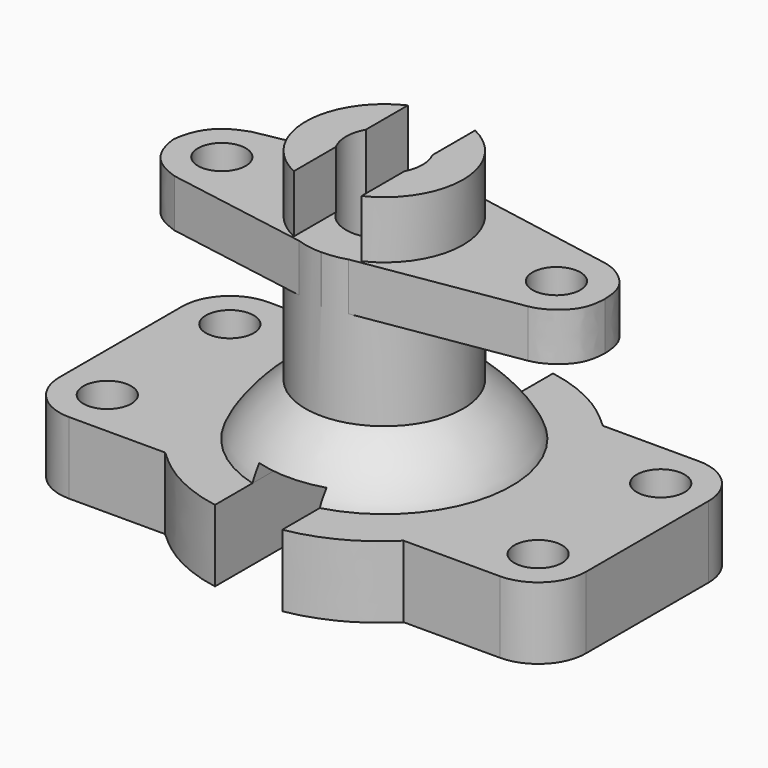
from build123d import *

# Parameters (mm, degrees)
F1_DEPTH  = 150
F2_R      = 100
F3_R      = 100
F4_R      = 100
F5_R      = 100
F6_R      = 50
F6_W      = 140.4859647155
F6_H      = 520
F6_H_2    = 39.2821230811
F6_H_3    = 46.7312682828
F7_DEPTH  = 150
F11_DEPTH = 30
F12_W     = 140.4859647155
F12_H     = 552.6287908551
F12_H_2   = 21.1866145137
F13_DEPTH = 25
F14_R     = 164.5018596362
F15_DEPTH = 500
F16_W     = 140.9460157156
F16_H     = 576.6842067242
F17_DEPTH = 120
F19_DEPTH = 100
F20_R     = 50
F21_DEPTH = 100
F22_R     = 80
F23_DEPTH = 600


with BuildPart() as f1:
    # F0 (on Top) → F1 (new body)
    with BuildSketch(Plane.XY):
        Polygon((-255.04347682, 304.850508936), (-555.8274231851, 304.850508936), (-555.8274231851, -215.149491064), (-255.04347682, -215.149491064), (-76.0704055429, -215.149491064), (64.4155591726, -215.149491064), (243.3886304498, -215.149491064), (544.1725768149, -215.149491064), (544.1725768149, 304.850508936), (243.3886304498, 304.850508936), (64.4155591726, 304.850508936), (-76.0704055429, 304.850508936), align=None)
        with BuildLine():
            add(Edge.make_bspline(
                [(-76.0704055429, 398.3130455017), (-111.1650615931, 392.6026821136), (-174.2262606106, 368.6970989499), (-217.5068408251, 339.1989171505), (-255.04347682, 304.850508936)],
                knots=[0, 0, 0, 0, 0.4864834978, 1, 1, 1, 1], degree=3))
            Line((-255.04347682, 304.850508936), (-76.0704055429, 304.850508936))
            Line((-76.0704055429, 304.850508936), (-76.0704055429, 398.3130455017))
        make_face()
        with BuildLine():
            Line((-76.0704055429, -215.149491064), (-255.04347682, -215.149491064))
            add(Edge.make_bspline(
                [(-76.0704055429, -308.6120276296), (-111.1650615931, -302.9016642416), (-174.2262606106, -278.9960810778), (-217.5068408251, -249.4978992784), (-255.04347682, -215.149491064)],
                knots=[0, 0, 0, 0, 0.4864834978, 1, 1, 1, 1], degree=3))
            Line((-76.0704055429, -308.6120276296), (-76.0704055429, -215.149491064))
        make_face()
        with BuildLine():
            Line((64.4155591726, 398.3130455017), (64.4155591726, 304.850508936))
            Line((64.4155591726, 304.850508936), (243.3886304498, 304.850508936))
            add(Edge.make_bspline(
                [(64.4155591726, 398.3130455017), (99.5102152228, 392.6026821136), (162.5714142404, 368.6970989499), (205.8519944549, 339.1989171505), (243.3886304498, 304.850508936)],
                knots=[0, 0, 0, 0, 0.4864834978, 1, 1, 1, 1], degree=3))
        make_face()
        with BuildLine():
            Line((243.3886304498, -215.149491064), (64.4155591726, -215.149491064))
            Line((64.4155591726, -215.149491064), (64.4155591726, -308.6120276296))
            add(Edge.make_bspline(
                [(64.4155591726, -308.6120276296), (99.5102152228, -302.9016642416), (162.5714142404, -278.9960810778), (205.8519944549, -249.4978992784), (243.3886304498, -215.149491064)],
                knots=[0, 0, 0, 0, 0.4864834978, 1, 1, 1, 1], degree=3))
        make_face()
    extrude(amount=F1_DEPTH)

    # F2
    f2_edges = [f1.edges().sort_by_distance(p)[0] for p in [
        (-555.827423, -215.149491, 75),
    ]]
    fillet(f2_edges, radius=F2_R)

    # F3
    f3_edges = [f1.edges().sort_by_distance(p)[0] for p in [
        (-555.827423, 304.850509, 75),
    ]]
    fillet(f3_edges, radius=F3_R)

    # F4
    f4_edges = [f1.edges().sort_by_distance(p)[0] for p in [
        (544.172577, 304.850509, 75),
    ]]
    fillet(f4_edges, radius=F4_R)

    # F5
    f5_edges = [f1.edges().sort_by_distance(p)[0] for p in [
        (544.172577, -215.149491, 75),
    ]]
    fillet(f5_edges, radius=F5_R)

    # F6 (on face) → F7 (cut)
    with BuildSketch(Plane.XY.offset(150)):
        with Locations((-455.8274231851, -115.149491064)):
            Circle(F6_R)
        with Locations((-455.8274231851, 204.850508936)):
            Circle(F6_R)
        with Locations((444.1725768149, 204.850508936)):
            Circle(F6_R)
        with Locations((444.1725768149, -115.149491064)):
            Circle(F6_R)
        with Locations((-5.8274231851, 44.850508936)):
            Rectangle(F6_W, F6_H)
        with Locations((-5.8274231851, 324.4915704766)):
            Rectangle(F6_W, F6_H_2)
        with Locations((-5.8274231851, -238.5151252054)):
            Rectangle(F6_W, F6_H_3)
    extrude(amount=-F7_DEPTH, mode=Mode.SUBTRACT)


with BuildPart() as f10:
    # F9 (on offset) → F10 (revolve)
    with BuildSketch(Plane.XZ.offset(-46)):
        with BuildLine():
            add(Edge.make_bspline(
                [(-170.576184988, 258.8557302952), (-198.9692002535, 247.1876442432), (-258.6858570576, 186.6178661585), (-272.3354101181, 149.9347686768)],
                knots=[0, 0, 0, 0, 149.0594370678, 149.0594370678, 149.0594370678, 149.0594370678], degree=3))
            Line((-272.3354101181, 149.9347686768), (-6.1521544121, 149.9347686768))
            Line((-6.1521544121, 149.9347686768), (-6.1521544121, 258.8557302952))
            Line((-6.1521544121, 258.8557302952), (-170.576184988, 258.8557302952))
        make_face()
    revolve(axis=Axis((-6.1521544121, 46, 204.395249486), (0, 0, 1)))

    # F6 (on face) → F11 (cut)
    with BuildSketch(Plane.XY.offset(150)):
        with Locations((-455.8274231851, -115.149491064)):
            Circle(F6_R)
        with Locations((-455.8274231851, 204.850508936)):
            Circle(F6_R)
        with Locations((444.1725768149, 204.850508936)):
            Circle(F6_R)
        with Locations((444.1725768149, -115.149491064)):
            Circle(F6_R)
        with Locations((-5.8274231851, 44.850508936)):
            Rectangle(F6_W, F6_H)
        with Locations((-5.8274231851, 324.4915704766)):
            Rectangle(F6_W, F6_H_2)
        with Locations((-5.8274231851, -238.5151252054)):
            Rectangle(F6_W, F6_H_3)
    extrude(amount=F11_DEPTH, mode=Mode.SUBTRACT)

    # F12 (on face) → F13 (cut)
    with BuildSketch(Plane.XY.offset(150)):
        with Locations((-5.8274231851, 56.1556639673)):
            Rectangle(F12_W, F12_H)
        with Locations((-5.8274231851, -230.7520387171)):
            Rectangle(F12_W, F12_H_2)
    extrude(amount=-F13_DEPTH, mode=Mode.SUBTRACT)

    # F14 (on face) → F15 (join)
    with BuildSketch(Plane(origin=(0, 0, 180), x_dir=(1, 0, 0), z_dir=(0, 0, -1))):
        with Locations((-6.1521544121, -46)):
            Circle(F14_R)
    extrude(amount=-F15_DEPTH)

    # F16 (on face) → F17 (cut)
    with BuildSketch(Plane.XY.offset(680)):
        with Locations((-5.5357143283, 38.3945852518)):
            Rectangle(F16_W, F16_H)
    extrude(amount=-F17_DEPTH, mode=Mode.SUBTRACT)

    # F18 (on face) → F19 (join)
    with BuildSketch(Plane.XY.offset(560)):
        with BuildLine():
            ThreePointArc((-76.0087221861, 194.932608124), (-71.1586390109, 197.1126029949), (-66.2406310646, 199.13470148))
            Line((-66.2406310646, 199.13470148), (-361.811041832, 142.5854861736))
            add(Edge.make_bspline(
                [(-361.811041832, 142.5854861736), (-379.9521342538, 136.153064008), (-417.6021453447, 119.6618540034), (-440.2464032173, 76.1652365327), (-443.6650574207, 42.4059182405)],
                knots=[0, 0, 0, 0, 0.4563088796, 1, 1, 1, 1], degree=3))
            add(Edge.make_bspline(
                [(-361.811041832, -57.7736496925), (-379.9521342538, -51.3412275269), (-417.6021453447, -34.8500175223), (-440.2464032173, 8.6465999484), (-443.6650574207, 42.4059182405)],
                knots=[0, 0, 0, 0, 0.4563088796, 1, 1, 1, 1], degree=3))
            Line((-361.811041832, -57.7736496925), (-60.1914490263, -109.3725087053))
            ThreePointArc((-60.1914490263, -109.3725087053), (-68.183712986, -106.3579586523), (-76.0087221861, -102.932608124))
            Line((-76.0087221861, -102.932608124), (-76.0087221861, 194.932608124))
        make_face()
        with BuildLine():
            Line((376.153409481, 141.4481401443), (50.8522174401, 200.3093108452))
            ThreePointArc((50.8522174401, 200.3093108452), (57.9640739697, 197.4924786313), (64.9372935295, 194.348077895))
            Line((64.9372935295, 194.348077895), (64.9372935295, -102.348077895))
            ThreePointArc((64.9372935295, -102.348077895), (54.9647832463, -106.7271480616), (44.724353476, -110.4367053121))
            Line((44.724353476, -110.4367053121), (376.153409481, -57.1924522519))
            add(Edge.make_bspline(
                [(376.153409481, -57.1924522519), (401.8360972404, -52.8410449624), (444.3782155693, -22.4764027045), (456.7823708057, 10.2454349399), (458.1390619278, 42.1278439462)],
                knots=[0, 0, 0, 0, 0.5069670176, 1, 1, 1, 1], degree=3))
            add(Edge.make_bspline(
                [(376.153409481, 141.4481401443), (401.8360972404, 137.0967328548), (444.3782155693, 106.732090597), (456.7823708057, 74.0102529526), (458.1390619278, 42.1278439462)],
                knots=[0, 0, 0, 0, 0.5069670176, 1, 1, 1, 1], degree=3))
        make_face()
        with BuildLine():
            ThreePointArc((-5.4699394357, 210.500445004), (-6.1521544121, 210.5018596362), (-6.8343693886, 210.500445004))
            Line((-6.8343693886, 210.500445004), (-66.2406310646, 199.13470148))
            ThreePointArc((-66.2406310646, 199.13470148), (-71.1586390109, 197.1126029949), (-76.0087221861, 194.932608124))
            Line((-76.0087221861, 194.932608124), (-76.0087221861, -102.932608124))
            ThreePointArc((-76.0087221861, -102.932608124), (-68.183712986, -106.3579586523), (-60.1914490263, -109.3725087053))
            Line((-60.1914490263, -109.3725087053), (-6.8343693886, -118.500445004))
            ThreePointArc((-6.8343693886, -118.500445004), (-6.1521544121, -118.5018596362), (-5.4699394357, -118.500445004))
            Line((-5.4699394357, -118.500445004), (44.724353476, -110.4367053121))
            ThreePointArc((44.724353476, -110.4367053121), (54.9647832463, -106.7271480616), (64.9372935295, -102.348077895))
            Line((64.9372935295, -102.348077895), (64.9372935295, 194.348077895))
            ThreePointArc((64.9372935295, 194.348077895), (57.9640739697, 197.4924786313), (50.8522174401, 200.3093108452))
            Line((50.8522174401, 200.3093108452), (-5.4699394357, 210.500445004))
        make_face()
    extrude(amount=-F19_DEPTH)

    # F20 (on face) → F21 (cut)
    with BuildSketch(Plane.XY.offset(560)):
        with Locations((-342.903257669, 42.8129918313)):
            Circle(F20_R)
        with Locations((357.0971113668, 41.4487451409)):
            Circle(F20_R)
    extrude(amount=-F21_DEPTH, mode=Mode.SUBTRACT)

    # F22 (on face) → F23 (cut)
    with BuildSketch(Plane.XY.offset(680)):
        with Locations((-6.1521544121, 46)):
            Circle(F22_R)
    extrude(amount=-F23_DEPTH, mode=Mode.SUBTRACT)


solid = Compound([f1.part, f10.part])
